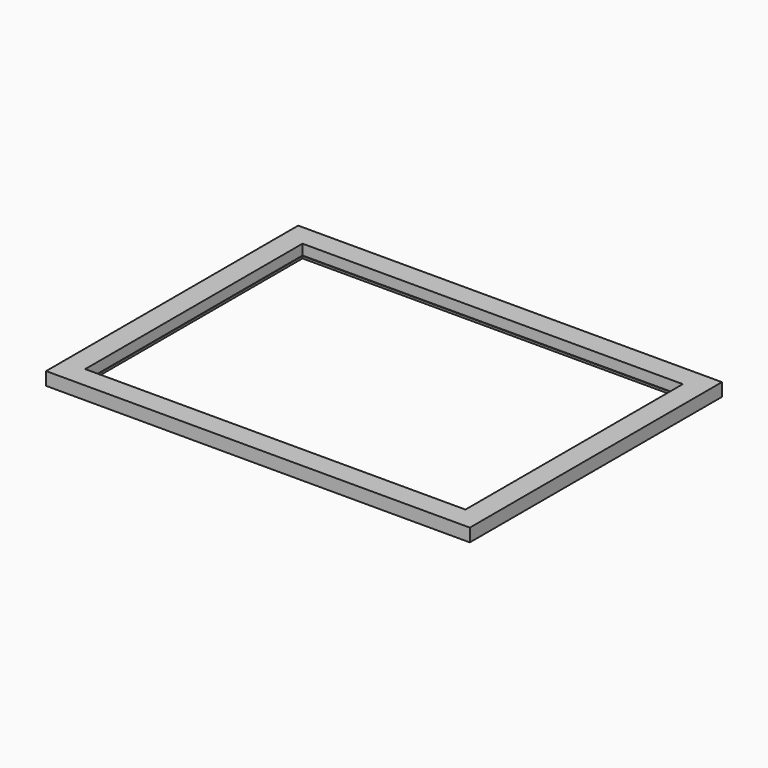
from build123d import *

# Parameters (mm, degrees)
F0_W     = 195
F0_H     = 145
F0_W_2   = 180
F0_H_2   = 130
F0_W_3   = 175
F0_H_3   = 125
F1_DEPTH = 5
F2_DEPTH = 1
F3_DEPTH = 0.2


with BuildPart() as f1:
    # F0 (on Top) → F1 (new body)
    with BuildSketch(Plane.XY):
        Rectangle(F0_W, F0_H)
        Rectangle(F0_W_2, F0_H_2, mode=Mode.SUBTRACT)
        Rectangle(F0_W_2, F0_H_2)
        Rectangle(F0_W_3, F0_H_3, mode=Mode.SUBTRACT)
    extrude(amount=F1_DEPTH)

    # F0 (on Top) → F2 (join)
    with BuildSketch(Plane.XY):
        Rectangle(F0_W, F0_H)
        Rectangle(F0_W_2, F0_H_2, mode=Mode.SUBTRACT)
        Rectangle(F0_W_2, F0_H_2)
        Rectangle(F0_W_3, F0_H_3, mode=Mode.SUBTRACT)
    extrude(amount=-F2_DEPTH)

    # F0 (on Top) → F3 (cut)
    with BuildSketch(Plane.XY):
        Rectangle(F0_W_2, F0_H_2)
        Rectangle(F0_W_3, F0_H_3, mode=Mode.SUBTRACT)
    extrude(amount=F3_DEPTH, mode=Mode.SUBTRACT)


solid = f1.part
